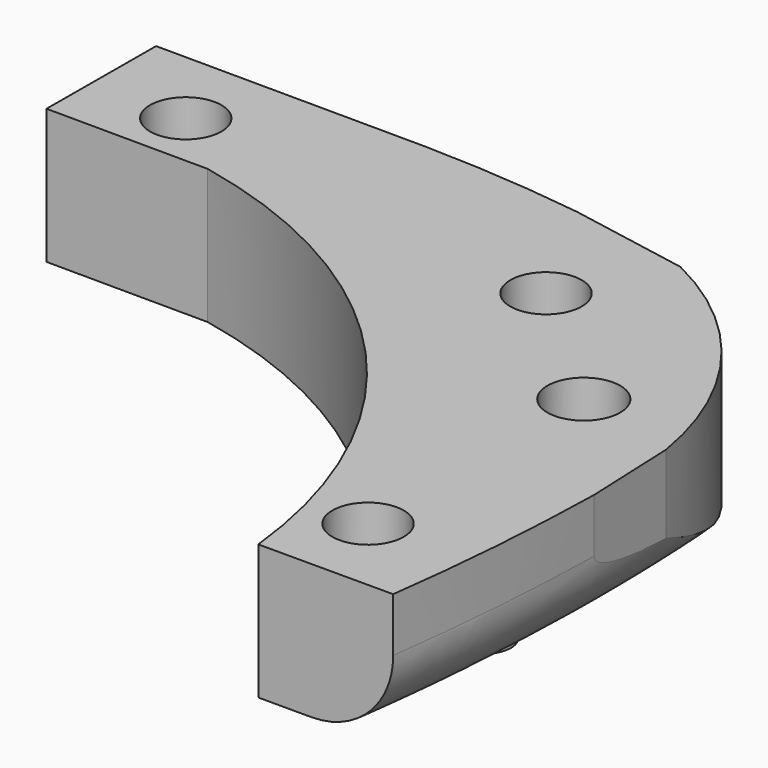
from build123d import *

# Parameters (mm, degrees)
F1_DEPTH    = 10
F2_R        = 2.65
F2_R_2      = 2.7
F3_DEPTH    = 10.001
F4_T2_ANGLE = 34.0182957269
F6_DEPTH    = 6
F7_R        = 1.99999
F8_T1_DEPTH = 13.9199888123


# Not quite as in the source:
# - a fillet or chamfer that OpenCascade refuses, or shapes differently, is made with other operations: its cross-section is extruded or revolved along the edge and cut away or added
# - a fillet or chamfer is up to 0.001 mm smaller than in the source, because OpenCascade refuses the exact size


with BuildPart() as f1:
    # F0 (on Top) → F1 (new body)
    with BuildSketch(Plane.XY):
        with BuildLine():
            Line((-33.6606874732, -11.2477834763), (-53.6606874732, -11.1477834763))
            Line((-53.6606874732, -11.1477834763), (-53.7111874732, -21.2477834763))
            Line((-53.7111874732, -21.2477834763), (-41.7113374704, -21.3077827264))
            ThreePointArc((-41.7113374704, -21.3077827264), (-20.1551088941, -33.6039887965), (-10, -56.2477834763))
            Line((-10, -56.2477834763), (0, -56.2477834763))
            ThreePointArc((0, -56.2477834763), (0.8963967025, -47.7664020072), (1.3093095262, -39.2477834763))
            Line((1.3093095262, -39.2477834763), (1.0172378853, -32.2477834763))
            ThreePointArc((1.0172378853, -32.2477834763), (-3.5776423647, -21.3591536143), (-12.6606874732, -13.7978391557))
            Line((-12.6606874732, -13.7978391557), (-21.6606874732, -12.1477834763))
            ThreePointArc((-21.6606874732, -12.1477834763), (-27.6471372828, -11.5171142711), (-33.6606874732, -11.2477834763))
        make_face()
    extrude(amount=F1_DEPTH)

    # F2 (on face) → F3 (cut, through all)
    with BuildSketch(Plane.XY.offset(10)):
        with Locations((-46.6606874732, -17.1477834763)):
            Circle(F2_R)
        with Locations((-16.6606874732, -21.2477834763)):
            Circle(F2_R)
        with Locations((-6.6606874732, -50.2477834763)):
            Circle(F2_R)
        with Locations((-6.6606874732, -30.2477834763)):
            Circle(F2_R_2)
    extrude(amount=-F3_DEPTH, mode=Mode.SUBTRACT)

    # F4: fillet of radius 6 on 1 edges, made by hand

    # F4_s1 → F4_t2 (revolve, cut)
    with BuildSketch(Plane(origin=(-32.1356329931, -81.9445924317, 0), x_dir=(0, 0, 1), z_dir=(-0.3650924394, -0.9309712727, 0))):
        with BuildLine():
            ThreePointArc((0, -18.8349622687), (1.7573593129, -23.0776029558), (6, -24.8349622687))
            Line((6, -24.8349622687), (6, -24.9549622687))
            Line((6, -24.9549622687), (-0.12, -24.9549622687))
            Line((-0.12, -24.9549622687), (-0.12, -18.8349622687))
            Line((-0.12, -18.8349622687), (0, -18.8349622687))
        make_face()
    revolve(axis=Axis((-148.6606874732, -36.2477834763, 0), (0, 0, 1)), revolution_arc=F4_T2_ANGLE, mode=Mode.SUBTRACT)

    # F5 (on face) → F6 (join)
    with BuildSketch(Plane.XY):
        with BuildLine():
            ThreePointArc((-19.6606874732, -34.1590258202), (-19.1967513982, -34.6993177477), (-18.7425076385, -35.2477834763))
            Line((-18.7425076385, -35.2477834763), (-9.6606874732, -35.2477834763))
            Line((-9.6606874732, -35.2477834763), (-9.6606874732, -31.2477834763))
            Line((-9.6606874732, -31.2477834763), (-19.6606874732, -31.2477834763))
            Line((-19.6606874732, -31.2477834763), (-19.6606874732, -34.1590258202))
        make_face()
    extrude(amount=-F6_DEPTH)

    # F7 (radius 2 in the source; OpenCascade refuses exactly that, so slightly less here)
    f7_edges = [f1.edges().sort_by_distance(p)[0] for p in [
        (-19.660687, -31.247783, -3),
        (-9.660687, -31.247783, -3),
        (-9.660687, -35.247783, -3),
    ]]
    fillet(f7_edges, radius=F7_R)

    # F8: fillet of radius 7 on 1 edges, made by hand

    # F8_s2 → F8_t1 (cut)
    with BuildSketch(Plane.XY.offset(-13.9199888123)):
        with BuildLine():
            ThreePointArc((-15.5745121135, -35.2477834763), (-18.3484354275, -34.6747072699), (-20.6681674701, -33.0493118901))
            ThreePointArc((-20.6681674701, -33.0493118901), (-19.6852521083, -34.1309546714), (-18.7425076385, -35.2477834763))
            Line((-18.7425076385, -35.2477834763), (-15.5745121135, -35.2477834763))
        make_face()
    extrude(amount=F8_T1_DEPTH, mode=Mode.SUBTRACT)


solid = f1.part
